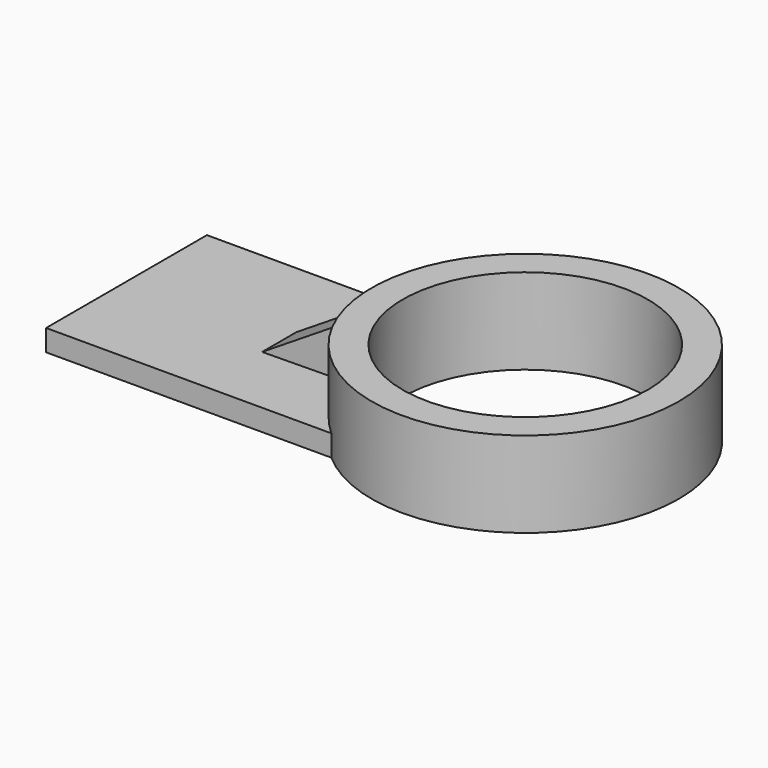
from build123d import *

# Parameters (mm, degrees)
F0_R     = 36.2745976669
F1_DEPTH = 25.4
F2_DEPTH = 6.35
F4_DEPTH = 12.7


# Not quite as in the source:
# - a length typed as a fraction of an inch, garbled in the dataset ("3 / 203.2 mm" for 3/8 in), is restored


with BuildPart() as f1:
    # F0 (on Top) → F1 (new body)
    with BuildSketch(Plane.XY):
        with BuildLine():
            ThreePointArc((-30.119665644, -34.1006480157), (18.7038816469, -41.4754537641), (45.4977851505, 0))
            ThreePointArc((45.4977851505, 0), (13.2923607222, 43.5127751359), (-37.7309519745, 25.4248641431))
            ThreePointArc((-37.7309519745, 25.4248641431), (-45.1303470765, -5.770634831), (-30.119665644, -34.1006480157))
        make_face()
        Circle(F0_R, mode=Mode.SUBTRACT)
    extrude(amount=F1_DEPTH)

    # F0 (on Top) → F2 (join)
    with BuildSketch(Plane.XY):
        with BuildLine():
            ThreePointArc((-30.119665644, -34.1006480157), (-45.1303470765, -5.770634831), (-37.7309519745, 25.4248641431))
            Line((-37.7309519745, 25.4248641431), (-114.592641592, 25.4248641431))
            Line((-114.592641592, 25.4248641431), (-114.592641592, -34.1006480157))
            Line((-114.592641592, -34.1006480157), (-30.119665644, -34.1006480157))
        make_face()
    extrude(amount=F2_DEPTH)


with BuildPart() as f4:
    # F3 (on Front) → F4 (new body)
    with BuildSketch(Plane.XZ):
        Polygon((-45.5851592124, 20.6049848348), (-67.7566081285, 6.6273342818), (-45.5851592124, 6.8683284335), align=None)
    extrude(amount=F4_DEPTH)


solid = Compound([f1.part, f4.part])
